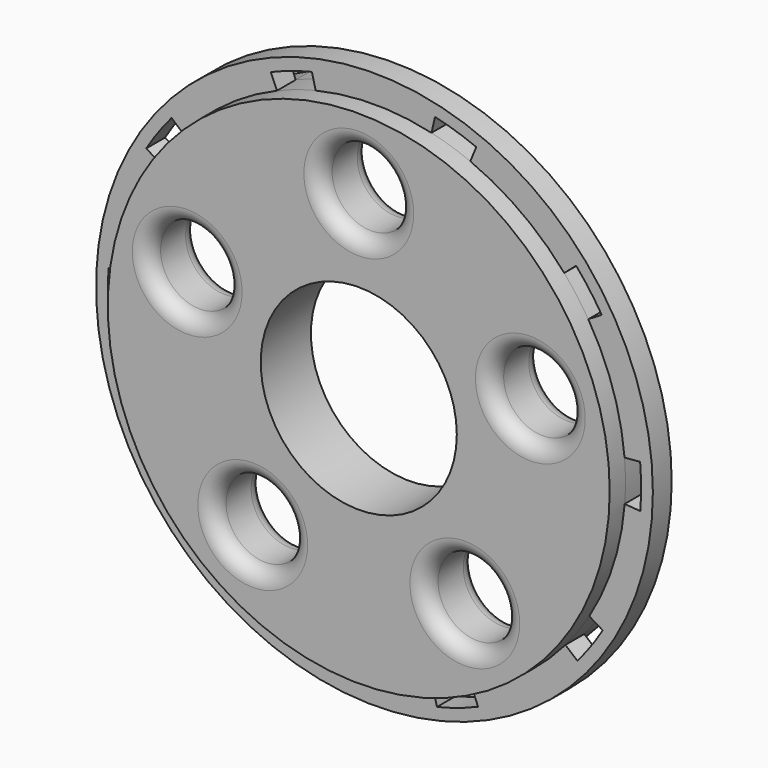
from build123d import *
from build123d import SkipClean  # not in build123d's __all__

# Parameters (mm, degrees)
F0_R          = 35.5
F1_DEPTH      = 4
F1_DEPTH_BACK = 4
F2_R          = 12.5
F3_DEPTH      = 25
F4_R          = 5
F5_DEPTH      = 25
F7_R          = 2
F8_R          = 36.3546739932
F8_R_2        = 32
F9_DEPTH      = 2.5
F10_R         = 42.2294694384
F10_R_2       = 32
F11_DEPTH     = 2.5
F13_DEPTH     = 25


# Not quite as in the source:
# - a feature names something its author has since deleted; it is built from what else it names


with BuildPart() as f1:
    # F0 (on Front) → F1 (new body, two sides)
    with BuildSketch(Plane.XZ) as f1_sk:
        Circle(F0_R)
    extrude(amount=-F1_DEPTH)
    extrude(f1_sk.sketch, amount=F1_DEPTH_BACK)

    # F2 (on face) → F3 (cut)
    with BuildSketch(Plane.XZ.offset(4)):
        Circle(F2_R)
    extrude(amount=-F3_DEPTH, mode=Mode.SUBTRACT)

    # F4 (on face) → F5 (cut)
    with BuildSketch(Plane.XZ.offset(4)):
        with Locations((0, 23)):
            Circle(F4_R)
        with Locations((-21.8742998748, 7.1073908706)):
            Circle(F4_R)
        with Locations((-13.5190608027, -18.6073908706)):
            Circle(F4_R)
        with Locations((13.5190608027, -18.6073908706)):
            Circle(F4_R)
        with Locations((21.8742998748, 7.1073908706)):
            Circle(F4_R)
    extrude(amount=-F5_DEPTH, mode=Mode.SUBTRACT)

    # F7
    f7_edges = [f1.edges().sort_by_distance(p)[0] for p in [
        (-5, -4, 23),
        (-26.8743, -4, 7.107391),
        (-18.519061, -4, -18.607391),
        (-26.8743, 4, 7.107391),
        (-18.519061, 4, -18.607391),
        (-5, 4, 23),
        (8.519061, -4, -18.607391),
        (8.519061, 4, -18.607391),
        (16.8743, -4, 7.107391),
        (16.8743, 4, 7.107391),
    ]]
    fillet(f7_edges, radius=F7_R)

    # F8 (on face) → F9 (cut)
    with BuildSketch(Plane.XZ.offset(4)):
        Circle(F8_R)
        Circle(F8_R_2, mode=Mode.SUBTRACT)
    extrude(amount=-F9_DEPTH, mode=Mode.SUBTRACT)

    # F10 (on face) → F11 (cut)
    with BuildSketch(Plane(origin=(0, 4, 0), x_dir=(-1, 0, 0), z_dir=(0, 1, 0))):
        Circle(F10_R)
        Circle(F10_R_2, mode=Mode.SUBTRACT)
    extrude(amount=-F11_DEPTH, mode=Mode.SUBTRACT)

    # F12 (on face) → F13 (cut)
    with BuildSketch(Plane.XZ.offset(1.5)):
        with BuildLine():
            ThreePointArc((7.2713328894, 31.1629221674), (9.7767280825, 30.4699128322), (12.2176076875, 29.5758357852))
            Line((12.2176076875, 29.5758357852), (12.981208168, 31.4243255218))
            ThreePointArc((12.981208168, 31.4243255218), (10.3877735876, 32.3742823842), (7.725791195, 33.1106048029))
            Line((7.725791195, 33.1106048029), (7.2713328894, 31.1629221674))
        make_face()
        with BuildLine():
            Line((-7.499987849, 31.1086833901), (-7.9687370895, 33.052976102))
            ThreePointArc((-7.9687370895, 33.052976102), (-10.6252403729, 32.2971247485), (-13.2116288258, 31.3281481063))
            Line((-13.2116288258, 31.3281481063), (-12.434474189, 29.4853158647))
            ThreePointArc((-12.434474189, 29.4853158647), (-10.0002262333, 30.3972938809), (-7.499987849, 31.1086833901))
        make_face()
        with BuildLine():
            Line((-24.3528429424, 20.7590712852), (-25.8748956263, 22.0565132405))
            ThreePointArc((-25.8748956263, 22.0565132405), (-27.5797736496, 19.8835631977), (-29.102655682, 17.5794036377))
            Line((-29.102655682, 17.5794036377), (-27.3907347595, 16.5453210707))
            ThreePointArc((-27.3907347595, 16.5453210707), (-25.9574340231, 18.7139418332), (-24.3528429424, 20.7590712852))
        make_face()
        with BuildLine():
            Line((-31.9037397545, 2.4801995243), (-33.8977234891, 2.6352119945))
            ThreePointArc((-33.8977234891, 2.6352119945), (-33.9997707942, -0.1248436771), (-33.8774572305, -2.8840755186))
            Line((-33.8774572305, -2.8840755186), (-31.8846656287, -2.7144240175))
            ThreePointArc((-31.8846656287, -2.7144240175), (-31.9997842769, -0.1174999314), (-31.9037397545, 2.4801995243))
        make_face()
        with BuildLine():
            Line((-27.2684923486, -16.7460241561), (-28.9727731204, -17.7926506658))
            ThreePointArc((-28.9727731204, -17.7926506658), (-27.4330111051, -20.0855645105), (-25.7122215694, -22.2459358528))
            Line((-25.7122215694, -22.2459358528), (-24.1997379476, -20.9373513909))
            ThreePointArc((-24.1997379476, -20.9373513909), (-25.8193045695, -18.9040607158), (-27.2684923486, -16.7460241561))
        make_face()
        with BuildLine():
            Line((-12.2176076875, -29.5758357852), (-12.981208168, -31.4243255218))
            ThreePointArc((-12.981208168, -31.4243255218), (-10.3877735876, -32.3742823842), (-7.725791195, -33.1106048029))
            Line((-7.725791195, -33.1106048029), (-7.2713328894, -31.1629221674))
            ThreePointArc((-7.2713328894, -31.1629221674), (-9.7767280825, -30.4699128322), (-12.2176076875, -29.5758357852))
        make_face()
        with BuildLine():
            Line((7.499987849, -31.1086833901), (7.9687370895, -33.052976102))
            ThreePointArc((7.9687370895, -33.052976102), (10.6252403729, -32.2971247485), (13.2116288258, -31.3281481063))
            Line((13.2116288258, -31.3281481063), (12.434474189, -29.4853158647))
            ThreePointArc((12.434474189, -29.4853158647), (10.0002262333, -30.3972938809), (7.499987849, -31.1086833901))
        make_face()
        with BuildLine():
            Line((24.3528429424, -20.7590712852), (25.8748956263, -22.0565132405))
            ThreePointArc((25.8748956263, -22.0565132405), (27.5797736496, -19.8835631977), (29.102655682, -17.5794036377))
            Line((29.102655682, -17.5794036377), (27.3907347595, -16.5453210707))
            ThreePointArc((27.3907347595, -16.5453210707), (25.9574340231, -18.7139418332), (24.3528429424, -20.7590712852))
        make_face()
        with BuildLine():
            Line((31.9037397545, -2.4801995243), (33.8977234891, -2.6352119945))
            ThreePointArc((33.8977234891, -2.6352119945), (33.9997707942, 0.1248436771), (33.8774572305, 2.8840755186))
            Line((33.8774572305, 2.8840755186), (31.8846656287, 2.7144240175))
            ThreePointArc((31.8846656287, 2.7144240175), (31.9997842769, 0.1174999314), (31.9037397545, -2.4801995243))
        make_face()
        with BuildLine():
            Line((27.2684923486, 16.7460241561), (28.9727731204, 17.7926506658))
            ThreePointArc((28.9727731204, 17.7926506658), (27.4330111051, 20.0855645105), (25.7122215694, 22.2459358528))
            Line((25.7122215694, 22.2459358528), (24.1997379476, 20.9373513909))
            ThreePointArc((24.1997379476, 20.9373513909), (25.8193045695, 18.9040607158), (27.2684923486, 16.7460241561))
        make_face()
    with SkipClean():  # cleaning this boolean's faces spoils the solid; the shape is the same uncleaned
        extrude(amount=-F13_DEPTH, mode=Mode.SUBTRACT)


solid = f1.part
